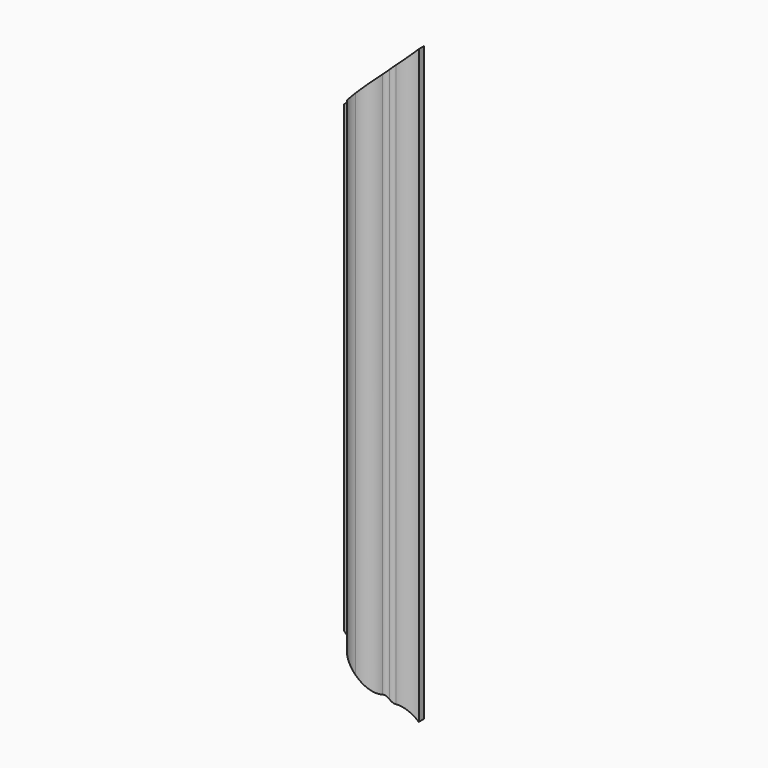
from build123d import *

# Parameters (mm, degrees)
F1_DEPTH = 146.05
F2_R     = 2.54
F3_R     = 2.54
F4_R     = 2.54
F6_DEPTH = 17.4635001
F8_DEPTH = 6.35


# Not quite as in the source:
# - ends of sketch curves that miss each other by under 0.0002 mm in the source are joined


with BuildPart() as f1:
    # F0 (on Top) → F1 (new body, symmetric)
    with BuildSketch(Plane.XY):
        with BuildLine():
            Line((15.875, 5.55625), (15.875, 8.73125))
            Line((15.875, 8.73125), (-15.875, 8.73125))
            Line((-15.875, 8.73125), (-15.875, -0.79375))
            Line((-15.875, -0.79375), (-12.7, -0.79375))
            ThreePointArc((-12.7, -0.79375), (-9.8710707302, -6.4481459867), (-3.9751, -8.73125))
            Line((-3.9751, -8.73125), (-3.96875, -8.73125))
            ThreePointArc((-3.96875, -8.73125), (1.9312218072, -6.4502821485), (4.7625, -0.79375))
            Line((4.7625, -0.79375), (7.9375, -0.79375))
            ThreePointArc((7.9375, -0.79375), (10.9883747468, 3.5285940665), (15.875, 5.55625))
        make_face()
    extrude(amount=F1_DEPTH, both=True)

    # F2
    f2_edges = [f1.edges().sort_by_distance(p)[0] for p in [
        (7.9375, -0.79375, 0),
    ]]
    fillet(f2_edges, radius=F2_R)

    # F3
    f3_edges = [f1.edges().sort_by_distance(p)[0] for p in [
        (-12.7, -0.79375, 0),
    ]]
    fillet(f3_edges, radius=F3_R)

    # F4
    f4_edges = [f1.edges().sort_by_distance(p)[0] for p in [
        (4.7625, -0.79375, 0),
    ]]
    fillet(f4_edges, radius=F4_R)

    # F5 (on face) → F6 (cut, through all)
    with BuildSketch(Plane(origin=(0, 8.73125, 0), x_dir=(-1, 0, 0), z_dir=(0, 1, 0))):
        Polygon((15.875, 146.05), (-15.875, 146.05), (15.875, 114.3), align=None)
        Polygon((15.875, -114.3), (-15.875, -146.05), (15.875, -146.05), align=None)
    extrude(amount=-F6_DEPTH, mode=Mode.SUBTRACT)

    # F7 (on face) → F8 (cut)
    with BuildSketch(Plane(origin=(0, 8.73125, 0), x_dir=(-1, 0, 0), z_dir=(0, 1, 0))):
        Polygon((9.525, 120.65), (9.525, -120.65), (15.875, -114.3), (15.875, 114.3), align=None)
    extrude(amount=-F8_DEPTH, mode=Mode.SUBTRACT)


solid = f1.part
